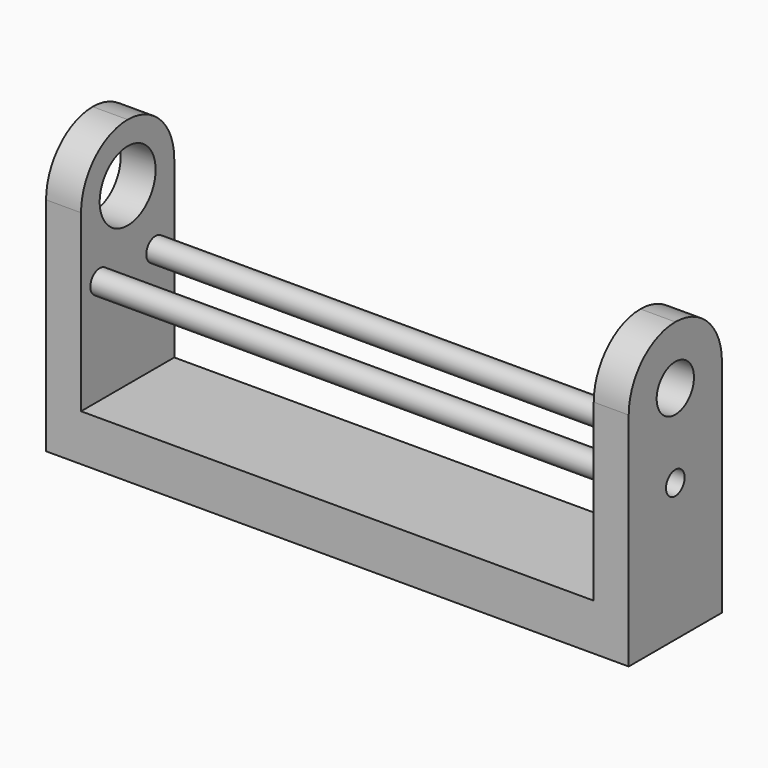
from build123d import *

# Parameters (mm, degrees)
F0_W      = 50
F0_H      = 10
F1_DEPTH  = 4
F2_W      = 3
F2_H      = 10
F3_DEPTH  = 20
F4_R      = 4.99999
F5_R      = 2
F6_DEPTH  = 25
F7_R      = 3
F8_DEPTH  = 25
F9_R      = 1
F10_DEPTH = 46
F11_R     = 1
F12_DEPTH = 25


# Not quite as in the source:
# - a fillet or chamfer is up to 0.001 mm smaller than in the source, because OpenCascade refuses the exact size


with BuildPart() as f1:
    # F0 (on Top) → F1 (new body)
    with BuildSketch(Plane.XY):
        Rectangle(F0_W, F0_H)
    extrude(amount=F1_DEPTH)

    # F2 (on face) → F3 (join)
    with BuildSketch(Plane.XY.offset(4)):
        with Locations((23.5, 0)):
            Rectangle(F2_W, F2_H)
        with Locations((-23.5, 0)):
            Rectangle(F2_W, F2_H)
    extrude(amount=F3_DEPTH)

    # F4 (radius 5 in the source; OpenCascade refuses exactly that, so slightly less here)
    f4_edges = [f1.edges().sort_by_distance(p)[0] for p in [
        (-23.5, -5, 24),
        (-23.5, 5, 24),
        (23.5, -5, 24),
        (23.5, 5, 24),
    ]]
    fillet(f4_edges, radius=F4_R)

    # F5 (on face) → F6 (cut)
    with BuildSketch(Plane.YZ.offset(25)):
        with Locations((0, 19)):
            Circle(F5_R)
    extrude(amount=-F6_DEPTH, mode=Mode.SUBTRACT)

    # F7 (on face) → F8 (cut)
    with BuildSketch(Plane.YZ.offset(-22)):
        with Locations((0, 19)):
            Circle(F7_R)
    extrude(amount=-F8_DEPTH, mode=Mode.SUBTRACT)

    # F9 (on face) → F10 (join)
    with BuildSketch(Plane.YZ.offset(-22)):
        with Locations((-3, 13)):
            Circle(F9_R)
        with Locations((3, 13)):
            Circle(F9_R)
    extrude(amount=F10_DEPTH)

    # F11 (on face) → F12 (cut)
    with BuildSketch(Plane(origin=(22, 0, 0), x_dir=(0, -1, 0), z_dir=(-1, 0, 0))):
        with Locations((0, 11.84)):
            Circle(F11_R)
    extrude(amount=-F12_DEPTH, mode=Mode.SUBTRACT)


solid = f1.part
